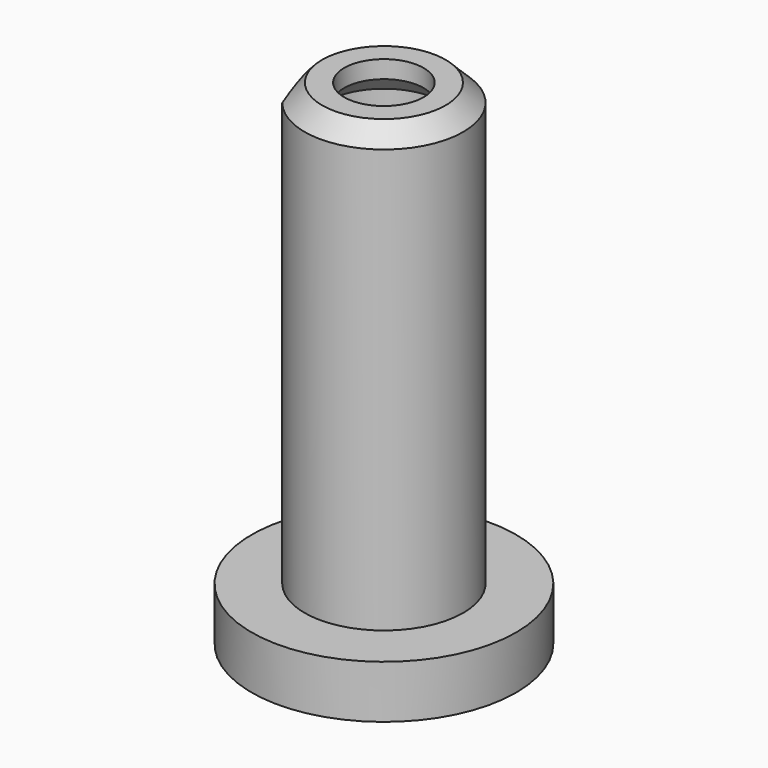
from build123d import *

# Parameters (mm, degrees)
F1_DEPTH       = 25
F0_R           = 7.5
F2_DEPTH       = 3
F3_D           = 6.5
F3_DEPTH       = 3.001
F4_D           = 4.5
F4_DEPTH       = 25
F4_CBORE_D     = 6.5
F4_CBORE_DEPTH = 23
F4_TIP         = 1.3519363928
F5_SIZE        = 0.99999


# Not quite as in the source:
# - a fillet or chamfer is up to 0.001 mm smaller than in the source, because OpenCascade refuses the exact size


with BuildPart() as f1:
    # F0 (on Top) → F1 (new body)
    with BuildSketch(Plane.XY):
        with BuildLine():
            Line((-3.5, 2.8284271247), (-3.5, -2.8284271247))
            ThreePointArc((-3.5, -2.8284271247), (4.5, 0), (-3.5, 2.8284271247))
        make_face()
    extrude(amount=F1_DEPTH)

    # F0 (on Top) → F2 (join)
    with BuildSketch(Plane.XY):
        Circle(F0_R)
        with BuildLine():
            ThreePointArc((-3.5, 2.8284271247), (4.5, 0), (-3.5, -2.8284271247))
            Line((-3.5, -2.8284271247), (-3.5, 2.8284271247))
        make_face(mode=Mode.SUBTRACT)
        with BuildLine():
            Line((-3.5, 2.8284271247), (-3.5, -2.8284271247))
            ThreePointArc((-3.5, -2.8284271247), (4.5, 0), (-3.5, 2.8284271247))
        make_face()
    extrude(amount=-F2_DEPTH)

    # F3 (through all, one way)
    with BuildSketch(Plane.XY):
        with Locations((0, 0)):
            Circle(F3_D / 2)
    extrude(amount=-F3_DEPTH, mode=Mode.SUBTRACT)

    # F4
    with Locations(Plane(origin=(0, 0, 0), x_dir=(1, 0, 0), z_dir=(0, 0, -1))):
        with Locations((0, 0)):
            CounterBoreHole(F4_D / 2, F4_CBORE_D / 2, F4_CBORE_DEPTH, depth=F4_DEPTH)
            with Locations((0, 0, -(F4_DEPTH + F4_TIP / 2))):  # 118° drill point
                Cone(0, F4_D / 2, F4_TIP, mode=Mode.SUBTRACT)

    # F5 (size 1 in the source; OpenCascade refuses exactly that, so slightly less here)
    f5_edges = [f1.edges().sort_by_distance(p)[0] for p in [
        (4.5, 0, 25),
        (-2.25, 0, 23),
    ]]
    chamfer(f5_edges, length=F5_SIZE)


solid = f1.part
